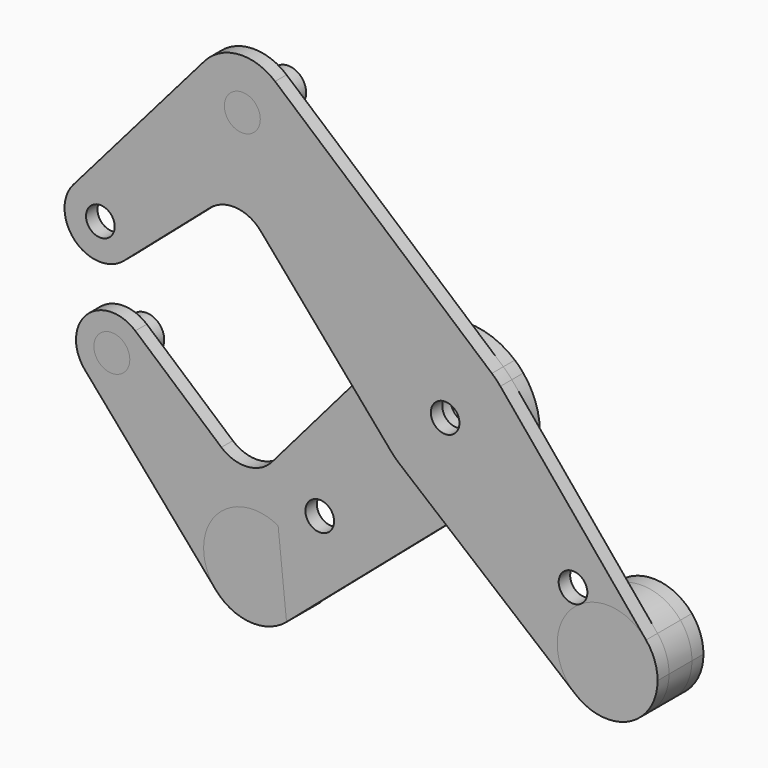
from build123d import *

# Parameters (mm, degrees)
F0_R     = 3.175
F0_R_2   = 3.9751
F1_DEPTH = 3.175
F2_DEPTH = 3.175
F4_R     = 3.175
F6_DEPTH = 9.525
F4_R_2   = 3.9751
F3_R     = 3.175
F3_R_2   = 3.9751


# Not quite as in the source:
# - a pattern or mirror of a feature is missing from the dataset's text; its kind, count and spacing are read off the source's solid


with BuildPart() as f1:
    # F0 (on Front) → F1 (new body)
    with BuildSketch(Plane.XZ):
        with BuildLine():
            ThreePointArc((-12.0356034274, 10.3518054047), (-1.190625, 15.8302885984), (10.3518054047, 12.0356034274))
            Line((10.3518054047, 12.0356034274), (-37.655016822, 53.3262030046))
            ThreePointArc((-37.655016822, 53.3262030046), (-34.8014845049, 49.5361241819), (-33.7887806053, 44.9012806053))
            ThreePointArc((-33.7887806053, 44.9012806053), (-48.7842347585, 34.4892527868), (-53.300199871, 52.1776678558))
            Line((-53.300199871, 52.1776678558), (-82.331405076, 18.6678036462))
            ThreePointArc((-82.331405076, 18.6678036462), (-73.5586383483, 20.9075469092), (-68.3946770291, 13.4703841816))
            ThreePointArc((-68.3946770291, 13.4703841816), (-69.1121208226, 10.1727039932), (-71.1347575644, 7.4711561347))
            Line((-71.1347575644, 7.4711561347), (-52.0843267669, 23.9754595323))
            ThreePointArc((-52.0843267669, 23.9754595323), (-46.2965222838, 25.8954961667), (-40.8511612346, 23.1508168672))
            Line((-40.8511612346, 23.1508168672), (-20.9391765456, 0))
            Line((-20.9391765456, 0), (-12.0356034274, 10.3518054047))
        make_face()
        with BuildLine():
            ThreePointArc((-68.3946770291, 13.4703841816), (-73.5586383483, 20.9075469092), (-82.331405076, 18.6678036462))
            ThreePointArc((-82.331405076, 18.6678036462), (-81.9448371048, 7.8577241059), (-71.1347575644, 7.4711561347))
            ThreePointArc((-71.1347575644, 7.4711561347), (-69.1121208226, 10.1727039932), (-68.3946770291, 13.4703841816))
        make_face()
        with Locations((-76.3321770291, 13.4703841816)):
            Circle(F0_R, mode=Mode.SUBTRACT)
        with BuildLine():
            ThreePointArc((-33.7887806053, 44.9012806053), (-34.8014845049, 49.5361241819), (-37.655016822, 53.3262030046))
            ThreePointArc((-37.655016822, 53.3262030046), (-45.7148756595, 55.9839571475), (-53.300199871, 52.1776678558))
            ThreePointArc((-53.300199871, 52.1776678558), (-48.7842347585, 34.4892527868), (-33.7887806053, 44.9012806053))
        make_face()
        with Locations((-44.9012806053, 44.9012806053)):
            Circle(F0_R, mode=Mode.SUBTRACT)
        with BuildLine():
            ThreePointArc((10.3518054047, -12.0356034274), (14.4282801435, -6.6212051093), (15.875, 0))
            ThreePointArc((15.875, 0), (14.9355142785, 5.3801522504), (12.2282550252, 10.1235074968))
            ThreePointArc((12.2282550252, 10.1235074968), (11.3304373246, 11.1192092809), (10.3518054047, 12.0356034274))
            ThreePointArc((10.3518054047, 12.0356034274), (-1.190625, 15.8302885984), (-12.0356034274, 10.3518054047))
            ThreePointArc((-12.0356034274, 10.3518054047), (-15.875, 0), (-12.0356034274, -10.3518054047))
            ThreePointArc((-12.0356034274, -10.3518054047), (-11.1192092809, -11.3304373246), (-10.1235074968, -12.2282550252))
            ThreePointArc((-10.1235074968, -12.2282550252), (0.1493607821, -15.87429735), (10.3518054047, -12.0356034274))
        make_face()
        Circle(F0_R_2, mode=Mode.SUBTRACT)
        with BuildLine():
            Line((0.1954344954, -20.7710836138), (10.3518054047, -12.0356034274))
            ThreePointArc((10.3518054047, -12.0356034274), (0.1493607821, -15.87429735), (-10.1235074968, -12.2282550252))
            Line((-10.1235074968, -12.2282550252), (0.1954344954, -20.7710836138))
        make_face()
        with BuildLine():
            ThreePointArc((-12.0356034274, -10.3518054047), (-15.875, 0), (-12.0356034274, 10.3518054047))
            Line((-12.0356034274, 10.3518054047), (-20.9391765456, 0))
            Line((-20.9391765456, 0), (-12.0356034274, -10.3518054047))
        make_face()
        with BuildLine():
            ThreePointArc((12.2282550252, 10.1235074968), (14.9355142785, 5.3801522504), (15.875, 0))
            ThreePointArc((15.875, 0), (14.4282801435, -6.6212051093), (10.3518054047, -12.0356034274))
            Line((10.3518054047, -12.0356034274), (0.1954344954, -20.7710836138))
            Line((0.1954344954, -20.7710836138), (28.8345692365, -44.4808030019))
            ThreePointArc((28.8345692365, -44.4808030019), (24.8320654939, -35.1980827435), (30.0059353765, -26.5136137301))
            ThreePointArc((30.0059353765, -26.5136137301), (37.6803721288, -24.9486796066), (44.4808030019, -28.8345692365))
            Line((44.4808030019, -28.8345692365), (12.2282550252, 10.1235074968))
        make_face()
        with BuildLine():
            ThreePointArc((31.490910058, -23.8257819975), (31.0949796313, -25.361163809), (30.0059353765, -26.5136137301))
            ThreePointArc((30.0059353765, -26.5136137301), (25.5368404848, -22.290400186), (31.490910058, -23.8257819975))
        make_face(mode=Mode.SUBTRACT)
        with BuildLine():
            ThreePointArc((47.0335244843, -35.9210244843), (46.3758844792, -32.154917909), (44.4808030019, -28.8345692365))
            ThreePointArc((44.4808030019, -28.8345692365), (37.6803721288, -24.9486796066), (30.0059353765, -26.5136137301))
            ThreePointArc((30.0059353765, -26.5136137301), (24.8320654939, -35.1980827435), (28.8345692365, -44.4808030019))
            ThreePointArc((28.8345692365, -44.4808030019), (40.650687385, -45.9767663811), (47.0335244843, -35.9210244843))
        make_face()
        with Locations((35.9210244843, -35.9210244843)):
            Circle(F0_R, mode=Mode.SUBTRACT)
        Circle(F0_R_2)
        Circle(F0_R, mode=Mode.SUBTRACT)
    extrude(amount=F1_DEPTH)


with BuildPart() as f2:
    # F0 (on Front) → F2 (new body)
    with BuildSketch(Plane.XZ):
        with BuildLine():
            Line((0.1954344954, -20.7710836138), (-10.1235074968, -12.2282550252))
            ThreePointArc((-10.1235074968, -12.2282550252), (-11.1192092809, -11.3304373246), (-12.0356034274, -10.3518054047))
            Line((-12.0356034274, -10.3518054047), (-20.9391765456, 0))
            Line((-20.9391765456, 0), (-40.8511612346, -23.1508168672))
            ThreePointArc((-40.8511612346, -23.1508168672), (-46.2965222838, -25.8954961667), (-52.0843267669, -23.9754595323))
            Line((-52.0843267669, -23.9754595323), (-71.1347575644, -7.4711561347))
            ThreePointArc((-71.1347575644, -7.4711561347), (-69.1121208226, -10.1727039932), (-68.3946770291, -13.4703841816))
            ThreePointArc((-68.3946770291, -13.4703841816), (-73.5586383483, -20.9075469092), (-82.331405076, -18.6678036462))
            Line((-82.331405076, -18.6678036462), (-53.300199871, -52.1776678558))
            ThreePointArc((-53.300199871, -52.1776678558), (-48.7842347585, -34.4892527868), (-33.7887806053, -44.9012806053))
            ThreePointArc((-33.7887806053, -44.9012806053), (-34.8014845049, -49.5361241819), (-37.655016822, -53.3262030046))
            Line((-37.655016822, -53.3262030046), (0.1954344954, -20.7710836138))
        make_face()
        with Locations((-30.2993841525, -30.2993841525)):
            Circle(F0_R, mode=Mode.SUBTRACT)
        with BuildLine():
            ThreePointArc((-53.300199871, -52.1776678558), (-45.7148756595, -55.9839571475), (-37.655016822, -53.3262030046))
            ThreePointArc((-37.655016822, -53.3262030046), (-34.8014845049, -49.5361241819), (-33.7887806053, -44.9012806053))
            ThreePointArc((-33.7887806053, -44.9012806053), (-48.7842347585, -34.4892527868), (-53.300199871, -52.1776678558))
        make_face()
        with Locations((-44.9012806053, -44.9012806053)):
            Circle(F0_R, mode=Mode.SUBTRACT)
        with BuildLine():
            ThreePointArc((-71.1347575644, -7.4711561347), (-81.9448371048, -7.8577241059), (-82.331405076, -18.6678036462))
            ThreePointArc((-82.331405076, -18.6678036462), (-73.5586383483, -20.9075469092), (-68.3946770291, -13.4703841816))
            ThreePointArc((-68.3946770291, -13.4703841816), (-69.1121208226, -10.1727039932), (-71.1347575644, -7.4711561347))
        make_face()
        with Locations((-76.3321770291, -13.4703841816)):
            Circle(F0_R, mode=Mode.SUBTRACT)
        with BuildLine():
            ThreePointArc((-12.0356034274, -10.3518054047), (-15.875, 0), (-12.0356034274, 10.3518054047))
            Line((-12.0356034274, 10.3518054047), (-20.9391765456, 0))
            Line((-20.9391765456, 0), (-12.0356034274, -10.3518054047))
        make_face()
        with BuildLine():
            Line((0.1954344954, -20.7710836138), (10.3518054047, -12.0356034274))
            ThreePointArc((10.3518054047, -12.0356034274), (0.1493607821, -15.87429735), (-10.1235074968, -12.2282550252))
            Line((-10.1235074968, -12.2282550252), (0.1954344954, -20.7710836138))
        make_face()
        with BuildLine():
            ThreePointArc((10.3518054047, -12.0356034274), (14.4282801435, -6.6212051093), (15.875, 0))
            ThreePointArc((15.875, 0), (14.9355142785, 5.3801522504), (12.2282550252, 10.1235074968))
            ThreePointArc((12.2282550252, 10.1235074968), (11.3304373246, 11.1192092809), (10.3518054047, 12.0356034274))
            ThreePointArc((10.3518054047, 12.0356034274), (-1.190625, 15.8302885984), (-12.0356034274, 10.3518054047))
            ThreePointArc((-12.0356034274, 10.3518054047), (-15.875, 0), (-12.0356034274, -10.3518054047))
            ThreePointArc((-12.0356034274, -10.3518054047), (-11.1192092809, -11.3304373246), (-10.1235074968, -12.2282550252))
            ThreePointArc((-10.1235074968, -12.2282550252), (0.1493607821, -15.87429735), (10.3518054047, -12.0356034274))
        make_face()
        Circle(F0_R_2, mode=Mode.SUBTRACT)
    extrude(amount=-F2_DEPTH)


with BuildPart() as f6:
    # F4 (on face) → F6 (new body, through all)
    with BuildSketch(Plane.XZ):
        with BuildLine():
            Line((-37.655016822, -53.3262030046), (-39.5136587319, -35.1821660984))
            ThreePointArc((-39.5136587319, -35.1821660984), (-53.5313876726, -37.9006443302), (-53.300199871, -52.1776678558))
            ThreePointArc((-53.300199871, -52.1776678558), (-45.7148756595, -55.9839571475), (-37.655016822, -53.3262030046))
        make_face()
        with Locations((-44.9012806053, -44.9012806053)):
            Circle(F4_R, mode=Mode.SUBTRACT)
        with Locations((-44.9012806053, -44.9012806053)):
            Circle(F4_R)
    extrude(amount=-F6_DEPTH)


with BuildPart() as f6b:
    # F4 (on face) → F6, piece 2 (new body, through all)
    with BuildSketch(Plane.XZ):
        with Locations((-76.3321770291, -13.4703841816)):
            Circle(F4_R_2)
        with Locations((-76.3321770291, -13.4703841816)):
            Circle(F4_R, mode=Mode.SUBTRACT)
        with Locations((-76.3321770291, -13.4703841816)):
            Circle(F4_R)
    extrude(amount=-F6_DEPTH)


with BuildPart() as f6c:
    # F3 (on face) → F6, piece 3 (new body, through all)
    with BuildSketch(Plane.XZ.offset(3.175)):
        with BuildLine():
            ThreePointArc((28.8345692365, -44.4808030019), (40.650687385, -45.9767663811), (47.0335244843, -35.9210244843))
            ThreePointArc((47.0335244843, -35.9210244843), (46.3758844792, -32.154917909), (44.4808030019, -28.8345692365))
            ThreePointArc((44.4808030019, -28.8345692365), (37.6803722871, -24.9486796319), (30.005935648, -26.5136135595))
            ThreePointArc((30.005935648, -26.5136135595), (24.8320655044, -35.1980825835), (28.8345692365, -44.4808030019))
        make_face()
        with Locations((35.9210244843, -35.9210244843)):
            Circle(F3_R, mode=Mode.SUBTRACT)
        with Locations((35.9210244843, -35.9210244843)):
            Circle(F3_R)
    extrude(amount=-F6_DEPTH)

    # F6_3_copies: F6c across plane


with BuildPart() as f6d:
    # F3 (on face) → F6, piece 4 (new body, through all)
    with BuildSketch(Plane.XZ.offset(3.175)):
        with Locations((-44.9012806053, 44.9012806053)):
            Circle(F3_R_2)
        with Locations((-44.9012806053, 44.9012806053)):
            Circle(F3_R, mode=Mode.SUBTRACT)
        with Locations((-44.9012806053, 44.9012806053)):
            Circle(F3_R)
    extrude(amount=-F6_DEPTH)

    # F6_4_copies: F6d across plane


with BuildPart() as f6c_1:
    add(f6c.part)
    add(f6c.part.mirror(Plane.ZX.offset(3.175)))


with BuildPart() as f6d_1:
    add(f6d.part)
    add(f6d.part.mirror(Plane.ZX.offset(3.175)))


solid = Compound([f1.part, f2.part, f6.part, f6b.part, f6c_1.part, f6d_1.part])
